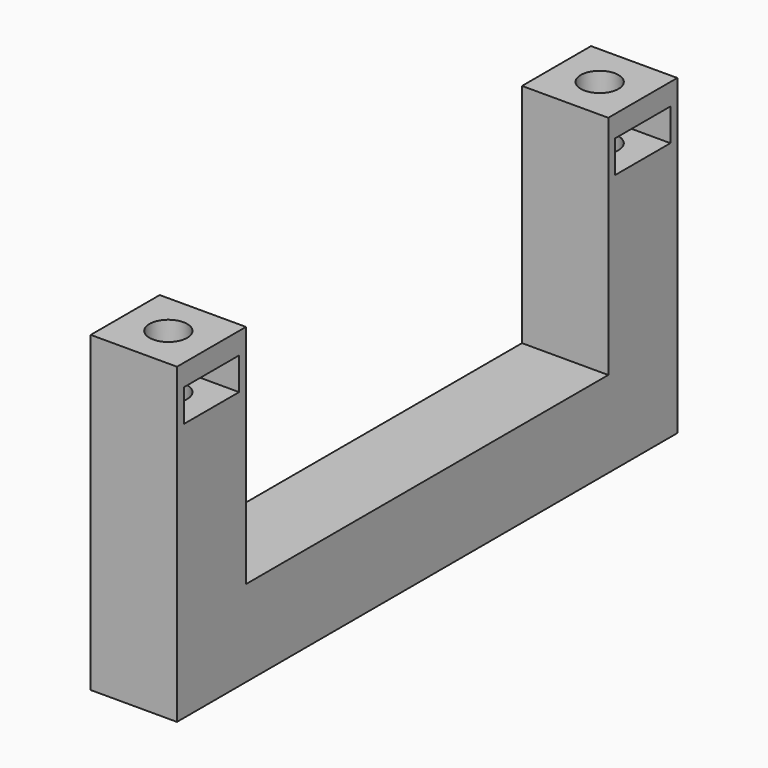
from build123d import *

# Parameters (mm, degrees)
F1_W     = 8
F1_H     = 58
F2_DEPTH = 8
F3_W     = 8
F3_H     = 8
F4_DEPTH = 21
F5_R     = 1.75
F6_DEPTH = 30
F7_W     = 6.4
F7_H     = 3
F8_DEPTH = 25
F9_DEPTH = 30


# Not quite as in the source:
# - a feature names something its author has since deleted; it is built from what else it names


with BuildPart() as f2:
    # F1 (on Top) → F2 (new body)
    with BuildSketch(Plane.XY):
        Rectangle(F1_W, F1_H)
    extrude(amount=F2_DEPTH)

    # F3 (on face) → F4 (join)
    with BuildSketch(Plane.XY.offset(8)):
        with Locations((0, 25)):
            Rectangle(F3_W, F3_H)
        with Locations((0, -25)):
            Rectangle(F3_W, F3_H)
    extrude(amount=F4_DEPTH)

    # F5 (on face) → F6 (cut)
    with BuildSketch(Plane.XY.offset(29)):
        with Locations((0, 25)):
            Circle(F5_R)
    extrude(amount=-F6_DEPTH, mode=Mode.SUBTRACT)

    # F7 (on face) → F8 (cut)
    with BuildSketch(Plane(origin=(-4, 0, 0), x_dir=(0, -1, 0), z_dir=(-1, 0, 0))):
        with Locations((-25, 25.5)):
            Rectangle(F7_W, F7_H)
        with Locations((25, 25.5)):
            Rectangle(F7_W, F7_H)
    extrude(amount=-F8_DEPTH, mode=Mode.SUBTRACT)

    # F5 (on face) → F9 (cut)
    with BuildSketch(Plane.XY.offset(29)):
        with Locations((0, 25)):
            Circle(F5_R)
        with Locations((0, -25)):
            Circle(F5_R)
    extrude(amount=-F9_DEPTH, mode=Mode.SUBTRACT)


solid = f2.part
